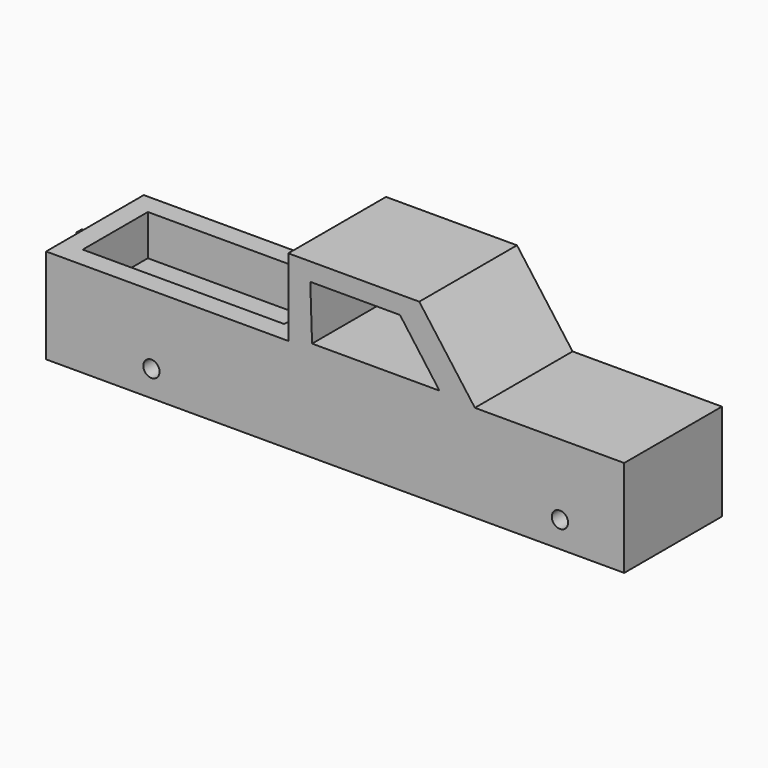
from build123d import *

# Parameters (mm, degrees)
F0_R         = 2
F1_DEPTH     = 30
F2_TEXT_SIZE = 24.7036313845
F3_DEPTH     = 3
F4_W         = 49.5014601144
F4_H         = 20.0000002235
F5_DEPTH     = 10


# Not quite as in the source:
# - Text() gives the source's letters only with a copy of the font that has no kerning and outlines rounded to 1/6400 em; it was checked with that copy


with BuildPart() as f1:
    # F0 (on Front) → F1 (new body)
    with BuildSketch(Plane.XZ):
        Polygon((-914.5565155536, -95.0207411238), (-914.5565155536, -118.3569370912), (-772.5318547696, -118.3569370912), (-772.5318547696, -94.5799879281), (-809.2168920938, -94.5799879281), (-822.8801884156, -76.0684222772), (-855.0550556628, -76.0684222772), (-855.0550556628, -95.0207411238), align=None)
        with Locations((-888.6798573162, -111.9817250662)):
            Circle(F0_R, mode=Mode.SUBTRACT)
        with Locations((-788.3255513832, -111.9817250662)):
            Circle(F0_R, mode=Mode.SUBTRACT)
        Polygon((-849.2135225355, -93.7031257968), (-849.6542862797, -80.4805773963), (-827.6167319838, -80.4805773963), (-817.9201827769, -93.7031257968), align=None, mode=Mode.SUBTRACT)
    extrude(amount=F1_DEPTH)

    # F2 (on face) → F3 (join)
    with BuildSketch(Plane(origin=(-914.5565155536, 0, 0), x_dir=(0, -1, 0), z_dir=(-1, 0, 0))):
        with Locations((6.6465693526, -115.9540638328)):
            Text('$', F2_TEXT_SIZE, font='Open Sans', font_style=FontStyle.BOLDITALIC, text_align=(TextAlign.LEFT, TextAlign.BOTTOM))
    extrude(amount=F3_DEPTH)

    # F4 (on face) → F5 (cut)
    with BuildSketch(Plane.XY.offset(-95.0207411238)):
        with Locations((-884.8057856082, -15)):
            Rectangle(F4_W, F4_H)
    extrude(amount=-F5_DEPTH, mode=Mode.SUBTRACT)


solid = f1.part
